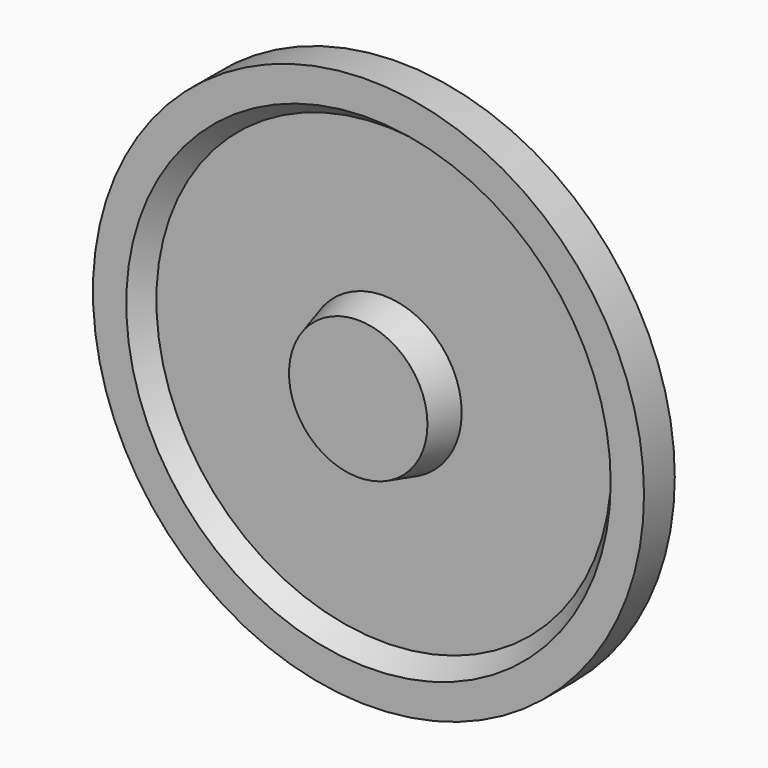
from build123d import *

# Parameters (mm, degrees)
F0_R     = 430
F1_DEPTH = 30
F2_R     = 385
F2_R_2   = 100
F3_DEPTH = 30
F4_DEPTH = 20


# Not quite as in the source:
# - a fillet or chamfer that OpenCascade refuses, or shapes differently, is made with other operations: its cross-section is extruded or revolved along the edge and cut away or added


with BuildPart() as f1:
    # F0 (on Front) → F1 (new body, symmetric)
    with BuildSketch(Plane.XZ):
        Circle(F0_R)
    extrude(amount=F1_DEPTH, both=True)

    # F2 (on face) → F3 (cut)
    with BuildSketch(Plane.XZ.offset(30)):
        Circle(F2_R)
        Circle(F2_R_2, mode=Mode.SUBTRACT)
    extrude(amount=-F3_DEPTH, mode=Mode.SUBTRACT)

    # F4 (add): a face of the model
    f4_faces = [f1.faces().sort_by_distance(p)[0] for p in [
        (0, -30, 0),
    ]]
    extrude(f4_faces, amount=F4_DEPTH)

    # F5: chamfer of 80 x 21.4359353945 on 1 edges, made by hand


with BuildPart() as f5_tool2:
    # F5_s3 → F5_t4 (revolve)
    with BuildSketch(Plane.XY):
        Polygon((121.4359353945, 0), (100, -80), (100, 0), align=None)
    revolve(axis=Axis((0, 0, 0), (0, -1, 0)))

    split(bisect_by=Plane.XZ.offset(50), keep=Keep.BOTTOM)


with BuildPart() as f1_1:
    add(f1.part)

    # F5_t1: union F5_tool2
    add(f5_tool2.part)

    # F6: chamfer of 30 x 39.0967611852 on 1 edges, made by hand


with BuildPart() as f6_tool2:
    # F6_s3 → F6_t4 (revolve)
    with BuildSketch(Plane.XY):
        Polygon((385, -39.0967611852), (355, 0), (385, 0), align=None)
    revolve(axis=Axis((0, 0, 0), (0, -1, 0)))

    split(bisect_by=Plane.XZ.offset(30), keep=Keep.BOTTOM)


with BuildPart() as f1_2:
    add(f1_1.part)

    # F6_t1: union F6_tool2
    add(f6_tool2.part)


solid = f1_2.part
